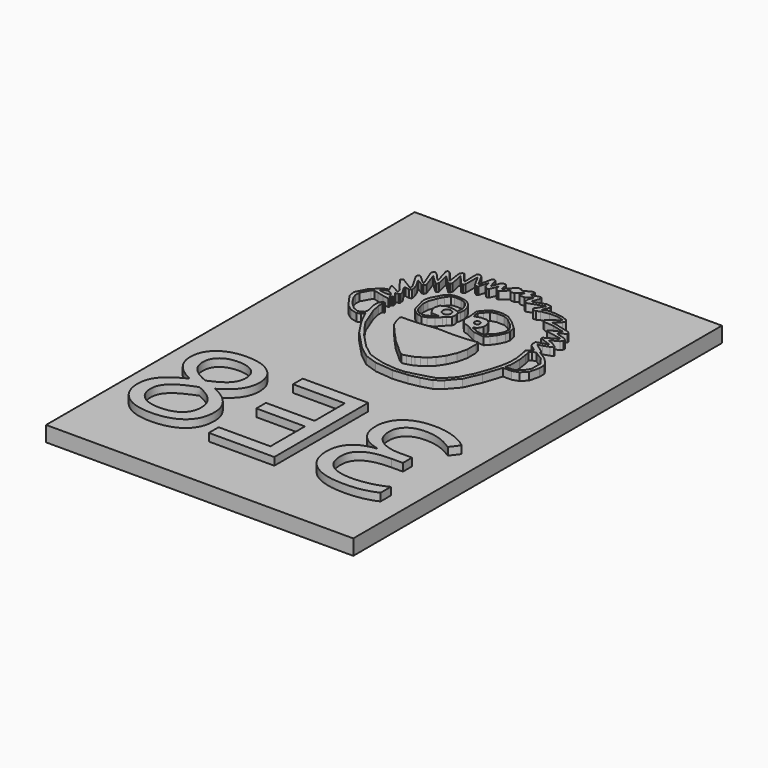
from build123d import *

# Parameters (mm, degrees)
F0_W         = 40
F0_H         = 60
F1_DEPTH     = 2
F2_TEXT_SIZE = 21.4073638846
F2_R         = 0.357844293
F2_R_2       = 0.5523242162
F3_DEPTH     = 3
F5_ANGLE     = 180


# Not quite as in the source:
# - Text() gives the source's letters only with a copy of the font that has no kerning and outlines rounded to 1/6400 em; it was checked with that copy


with BuildPart() as f1:
    # F0 (on Top) → F1 (new body)
    with BuildSketch(Plane.XY):
        Rectangle(F0_W, F0_H)
    extrude(amount=-F1_DEPTH)

    # F2 (on face) → F3 (join)
    with BuildSketch(Plane(origin=(0, 0, -2), x_dir=(1, 0, 0), z_dir=(0, 0, -1))):
        Polygon((-9.189459689, 13.5348810488), (-9.2555044294, 13.4181681694), (-10.3975787834, 12.584762522), (-10.4901792556, 12.3069606395), (-11.5087863133, 11.6587564023), (-12.1261237264, 11.0722858132), (-12.558260195, 10.424081576), (-12.558260195, 9.5906761614), (-12.2495910228, 8.3251342782), (-11.5705199614, 7.6151965092), (-10.7371147797, 7.3373945103), (-9.6259072498, 7.3373945103), (-8.8542347849, 4.9915125034), (-7.9282291308, 2.892565322), (-6.6935543046, 1.4726890856), (-5.7675486505, 0.7627512002), (-4.3785387725, 0.3614815557), (-3.0540523194, 0.0964602129), (-1.1776926304, -0.0722013741), (1.2046519941, 0.1597081916), (2.8912674561, 0.7289409311), (4.4724697172, 1.9728200184), (6.6861522309, 4.3129990715), (7.9932792969, 6.3158551108), (8.6257604807, 7.6018992019), (8.8155044168, 8.0235530529), (9.1317452416, 7.6440645987), (9.5744810924, 7.4543205462), (10.4388723075, 7.6862299954), (11.2610969618, 8.2765453168), (12.504976049, 10.0264091649), (12.6525543555, 10.8907999144), (11.8935786113, 12.3665881017), (11.2610969618, 12.9498689109), (10.7947986498, 13.3703084336), (10.322515659, 13.5592216299), (10.1808307618, 13.5592216299), (10.5303207338, 14.3337667593), (10.4219816507, 14.382651481), (9.6046447679, 13.9559403667), (9.3968396932, 13.7670267047), (9.1512517929, 13.7670267047), (9.302383095, 14.1920818621), (9.9541338086, 14.9855184042), (10.690847218, 15.9883339563), (10.3991904993, 16.2025981001), (8.8826266974, 15.2650455618), (8.7546797395, 15.3171446779), (8.8031513542, 15.6388244265), (9.8634593114, 17.4857479194), (9.8634593114, 17.788693183), (9.7230512574, 17.901346893), (9.4896217733, 17.8499919036), (8.4695348441, 16.8905964726), (8.369159691, 16.8905964726), (8.369159691, 17.0469944039), (9.1667303741, 19.0665655443), (9.1088505387, 19.4099162379), (8.9197883308, 19.5366152236), (8.4184741527, 19.1508362674), (7.6857789345, 18.2866071024), (7.5817767456, 18.2866071024), (8.1641504466, 20.2886032545), (8.0856618397, 20.4456875705), (7.8857758008, 20.4456875705), (7.6628642082, 20.2821175241), (6.6878812313, 19.0010591083), (6.5792927444, 19.0010591083), (6.8152903504, 20.7254605972), (6.6392480321, 21.0585369402), (6.3932228759, 21.0585369402), (5.3943090997, 19.7659152233), (5.2640845924, 19.7659152233), (5.313896846, 20.6956349918), (5.313896846, 21.6737444186), (5.1276095137, 21.8378741899), (4.8515007756, 21.8378741899), (4.6102980077, 21.5991920465), (3.8448546938, 20.1628588745), (3.7508065251, 20.2129785426), (3.4124271869, 21.8915016064), (3.1986572239, 21.9903782615), (2.9369632639, 21.7998669156), (2.6018317248, 20.5726175242), (2.1652462119, 21.6910027572), (1.9358477779, 21.8655924288), (1.7066724058, 21.8655924288), (1.5171964578, 21.7885960498), (1.3179039042, 20.8237523818), (0.2019009071, 22.0263794669), (-0.2691809978, 22.0263794669), (-0.4132577642, 21.83376892), (-0.4132577642, 21.7485696682), (-1.608875541, 22.3511316487), (-1.8950914573, 22.2474922099), (-1.8950914573, 22.0347762713), (-1.7497865092, 21.5740854525), (-2.8787629754, 21.9201136985), (-3.0722433776, 21.8083903798), (-3.0722433776, 21.4888442912), (-2.7170588337, 20.5106659466), (-3.5181820467, 20.785703198), (-4.3758560978, 21.0735172638), (-4.9409458488, 20.9864795813), (-5.1119194441, 20.6827808776), (-4.6780330204, 19.7794426837), (-5.303144183, 20.0162407615), (-6.4228956662, 20.0162407615), (-7.4601017013, 19.8396731773), (-8.0307817161, 19.5844498136), (-8.24605041, 19.3033533776), (-8.0752160475, 18.9340774575), (-7.4343785718, 18.3960458868), (-7.3064819053, 18.2485942402), (-7.8894097433, 18.1528887385), (-9.8450260312, 17.662368589), (-10.0632274598, 17.4525257805), (-10.0632274598, 17.2588265174), (-9.2694286332, 16.7433804506), (-9.2694286332, 16.6299444297), (-10.3714356274, 16.3117515528), (-10.7497630716, 16.0429821023), (-10.7497630716, 15.8157105231), (-10.5060694814, 15.5290242889), (-9.5397301093, 15.0264118471), (-9.5050336868, 14.9278080696), (-10.1310964236, 14.7075108581), (-10.7881587073, 14.2786650592), (-10.8735991717, 14.1022418299), (-10.4952348931, 13.9190028099), (-9.6939068362, 13.6496204556), (-9.3001715914, 13.5726396599), align=None)
        Polygon((-11.3430276588, 11.3477747561), (-10.1665381417, 12.0761071936), (-9.7184592933, 11.9456195877), (-9.4817701802, 11.6775998519), (-9.6478203386, 10.9875624673), (-9.8202779964, 9.7875330736), (-9.8202779964, 8.327060719), (-9.6632728428, 7.6724917068), (-10.7016285956, 7.6724917068), (-11.5608099923, 8.2125865062), (-12.0227627531, 8.9787616068), (-12.0227627531, 10.4255544626), align=None, mode=Mode.SUBTRACT)
        Polygon((-9.2021089122, 11.8955987179), (-9.6259845495, 12.3817160399), (-8.7710965499, 13.0297950142), (-8.6582891718, 13.3749520079), (-8.6582891718, 13.83907801), (-10.1395716965, 14.2732391739), (-8.597789526, 14.8448477173), (-8.6321562603, 15.0500525394), (-8.8547609821, 15.1859855884), (-10.0988355736, 15.8662788417), (-10.1283473969, 16.0429821023), (-8.1280890927, 16.3770521664), (-8.0309549421, 16.4534951234), (-8.0309549421, 16.6605234751), (-9.3255780712, 17.2988389292), (-9.3255780712, 17.4198456713), (-9.1570152045, 17.4198456713), (-7.8610751853, 17.7576577896), (-6.6900786087, 17.8401813516), (-6.3190494739, 18.0482565099), (-6.3680035137, 18.2607452059), (-7.6723454595, 19.1558197745), (-7.7717725262, 19.3576820799), (-6.9919994176, 19.5941383624), (-5.8549048454, 19.5941383624), (-4.8648479469, 19.4219628954), (-4.4465760775, 19.1960696736), (-4.0711632073, 19.1960696736), (-3.8452727795, 19.4726091483), (-4.5987849198, 20.6631215894), (-2.4533390142, 19.9265553289), (-2.2179344278, 20.1073296973), (-2.2179344278, 20.7775569194), (-2.4591403605, 21.2532266278), (-2.3988887742, 21.3428641343), (-1.6459601075, 20.8367685461), (-0.9518933557, 20.8367685461), (-0.805045439, 21.019308702), (-1.0992089397, 21.5109431249), (-1.0195223922, 21.5961252013), (-0.2568764803, 20.8826814554), (0.2120201406, 20.8826814554), (0.3918342218, 21.084864498), (1.3117186418, 20.2667534956), (1.5177458217, 20.2667534956), (1.7740993453, 20.4911687085), (1.8939064275, 21.0153785208), (2.3163190735, 20.022345581), (2.6061288472, 19.9079726496), (2.9661786202, 20.2604381972), (3.1901370194, 20.9794900053), (3.5305980518, 19.7691152477), (3.7267443649, 19.6868980908), (4.0454394575, 19.8750336328), (4.8510113656, 21.3132694968), (4.8510113656, 19.3455516034), (5.0149255357, 19.1363542014), (5.2653525881, 19.1363542014), (6.4009947628, 20.4648094856), (6.0275097303, 18.7064808467), (6.1335333548, 18.439371013), (6.3022564091, 18.3301762351), (7.5222377591, 19.5092194387), (7.1205476224, 17.8356234589), (7.2578334175, 17.6346850255), (7.4274286553, 17.6533626997), (8.5592081696, 18.700335049), (7.8939602636, 16.7839758703), (8.0356148928, 16.4933296525), (8.2925388515, 16.4933296525), (9.1843039208, 17.0311035363), (8.6411859765, 16.0850601875), (8.3799024969, 15.3487844997), (8.3799024969, 15.0033094594), (8.5981579423, 14.851562553), (9.1992679909, 14.9908660584), (9.275292784, 14.8559425631), (9.1386919766, 14.569966928), (8.7421050221, 13.9571603992), (8.6583698094, 13.5250080982), (8.8074074983, 13.3611097605), (9.3035807758, 13.3611097605), (9.0055147111, 13.0921600991), (8.8328046649, 12.7726279804), (8.8328046649, 12.5881325127), (9.010963068, 12.5194479616), (9.1582264676, 12.3547840537), (8.9850995676, 12.1999519706), (8.9941497817, 11.9886224763), (9.1404642835, 11.9948884146), (9.803073287, 12.1258817287), (10.623873949, 12.3241915041), (11.2366292551, 12.4787016445), (11.5004207864, 12.2345046745), (12.1156934574, 11.1478128144), (12.1156934574, 10.499742222), (11.9622180164, 9.9955123057), (11.2739799469, 8.9259134745), (10.4609073996, 8.1680297059), (9.7701705917, 7.8610534453), (9.4209367335, 7.9873521951), (9.1028444394, 8.1669735861), (8.9708127007, 8.5515753505), (9.0506223887, 8.9722721511), (9.204881072, 9.5914580067), (9.2938465923, 10.2266588853), (9.2200411409, 10.6872914964), (9.0513963178, 10.9562481427), (8.8901601657, 11.0822765761), (8.7422074675, 11.0587918804), (8.550712645, 10.8786210091), (8.5594270304, 10.7580808596), (8.6830591708, 10.740066287), (8.7972700521, 10.740066287), (8.7972700521, 10.0910024391), (8.5443880334, 8.9049179712), (8.1242027618, 7.8653744328), (7.5713287033, 6.4385982311), (6.6861522309, 5.1533160055), (5.8046395816, 4.0356008009), (4.1952138226, 2.3478454584), (2.7228207718, 1.228510742), (1.6501371674, 0.8664269605), (0.5779551238, 0.5780266271), (-0.5085729254, 0.456186817), (-1.3347239774, 0.3945332625), (-2.4423787445, 0.4550575883), (-3.9167545811, 0.8341207774), (-5.5857125744, 1.3082342827), (-6.3966686912, 1.8832468101), (-7.3317719698, 2.9245937382), (-8.1612218246, 4.5228650467), (-8.7279576883, 6.1055318126), (-9.1673780307, 7.5941767915), (-9.3645185307, 8.7970305373), (-9.3645185307, 9.8288155766), (-9.2588907182, 10.5280371988), (-9.1195667237, 11.3835189165), (-9.0252330601, 11.7312156269), align=None, mode=Mode.SUBTRACT)
        Polygon((9.5603252399, 13.0371160598), (9.8843954429, 13.2374589936), (10.1001633256, 13.2788474345), (10.5121981278, 13.1799288699), (10.7520677075, 13.0064216116), (10.8275951743, 12.8346410253), (10.531334944, 12.7722703525), (9.9573207944, 12.6837141485), (9.5230515972, 12.7355725178), (9.3631798327, 12.8573070885), align=None, mode=Mode.SUBTRACT)
        with Locations((-18.0694767914, -22.5213780068)):
            Text('3E8', F2_TEXT_SIZE, font='Open Sans', text_align=(TextAlign.LEFT, TextAlign.BOTTOM))
        Polygon((-2.5932078324, 9.9378599459), (-4.112102285, 10.137641211), (-4.2508884408, 9.6318180346), (-4.2508884408, 8.2489791), (-3.955797486, 6.9681084621), (-3.4152941853, 5.7855350512), (-2.8328874223, 4.9387547094), (-2.2081053278, 4.3190151991), (-1.5957122278, 3.9136625034), (-1.1420036128, 3.6378370204), (-0.7815588806, 3.4961389517), (-0.2557291111, 3.3374889826), (0.1739065001, 3.2302179513), (0.3918342218, 3.2689726119), (0.9345906246, 3.6690056929), (1.5618625721, 4.2602275404), (2.2558979297, 4.8684978464), (2.7284528667, 5.3091954978), (3.2852092217, 5.9283885109), (4.0007627494, 6.6972817201), (4.986223571, 7.8703290689), (5.3999910988, 8.9265593467), (5.4964109249, 9.4528837269), (5.4245561287, 9.5860982453), (3.4754090402, 9.6415715431), (0.915597232, 9.9233951093), (-1.0267217485, 9.8763281619), align=None)
        Polygon((-2.1723929867, 16.6633695969), (-2.9941883013, 16.4811814809), (-3.9514216669, 15.8269059518), (-5.0155857653, 14.860567511), (-5.231388107, 13.9517475524), (-5.1017587148, 13.399936133), (-4.6788586378, 12.5413465918), (-4.2540195473, 11.9674516515), (-3.7715008557, 11.4688746305), (-2.396504434, 11.6344543712), (-1.0310241096, 12.3511621402), (-0.3819549065, 12.5246605509), (0.0503193105, 13.0420954571), (0.1300272515, 13.5537449875), (0.0762266672, 14.04781627), (0.2374199203, 15.27546613), (0.0723192743, 15.584278726), (-0.5345819709, 16.2360415467), (-1.0026836144, 16.5532434964), (-1.5766988117, 16.6633695969), align=None)
        Polygon((-0.1165750628, 14.7014631563), (-0.2550073159, 14.3229745933), (-0.8960224996, 14.5691278064), (-1.7319852095, 14.5779129722), (-2.2096724324, 14.2550364741), (-2.4325162713, 13.7577265174), (-2.4314398952, 13.1487640226), (-2.2201318834, 12.7197567978), (-1.9343653303, 12.4825419531), (-1.7724684049, 12.4704310344), (-1.7102676984, 12.396911499), (-1.7475855611, 12.2880044998), (-1.9782550708, 12.1759254159), (-2.3868969104, 11.9888812841), (-2.8266529162, 11.8933775136), (-3.1929185689, 11.8191562266), (-3.5008960013, 11.8640306079), (-4.4143565074, 12.7688402915), (-4.7701496706, 13.4648060099), (-4.9055812024, 14.2937785619), (-4.2933744453, 15.1877588266), (-3.2846883014, 15.9890929842), (-2.6140033342, 16.2630992615), (-1.6628834028, 16.2843315535), (-0.948295773, 16.0998616972), (-0.5027595516, 15.5382760474), (-0.1036080839, 15.070862011), align=None, mode=Mode.SUBTRACT)
        with Locations((-1.3843593961, 13.4500422188)):
            Circle(F2_R, mode=Mode.SUBTRACT)
        Polygon((1.3897048002, 14.2145490879), (1.4955032775, 13.7759790429), (1.3754680212, 13.3076755935), (1.44481593, 12.8413940453), (1.8575723907, 12.5119726778), (2.1335671581, 12.2160956868), (2.6614377666, 11.6326211625), (3.3475812915, 11.2160452315), (3.8980571944, 10.9935378329), (4.4548309333, 11.1040746467), (4.8146828003, 11.2889216886), (5.377754841, 11.7325027147), (5.6196123287, 12.3399951169), (5.7611589245, 13.0087415361), (5.9384720325, 13.6048718029), (5.9984850622, 14.1340073803), (5.7975801565, 14.8063533613), (5.3796086386, 15.5532209807), (5.1052549779, 16.0898835072), (4.737034712, 16.4509442308), (4.2349321693, 16.6769566619), (3.7436595112, 16.718240329), (3.1430330518, 16.6763922804), (2.4245591294, 16.4872872317), (1.8735466683, 16.0395660111), (1.5190454824, 15.4573375964), (1.3410480269, 14.7608806053), align=None)
        with Locations((2.4974290672, 13.3780193188)):
            Circle(F2_R_2, mode=Mode.SUBTRACT)
        Polygon((2.1974599613, 14.2699516052), (1.76839092, 14.1540587553), (1.6981912004, 14.913517856), (1.9746389398, 15.6931689614), (2.4569535553, 16.1895108083), (3.1037636027, 16.3751513371), (3.9679916035, 16.3960939878), (4.3323885575, 16.2988536665), (4.7341545969, 15.7875491911), (5.1109779551, 15.0563249969), (5.4991979077, 14.0314063662), (5.5442338735, 13.3672495046), (5.4463374354, 12.8113444568), (5.2143882885, 12.0803936058), (5.0212180167, 11.7598435515), (4.5457210317, 11.4395030448), (3.9612055216, 11.3684468576), (3.3014659229, 11.6317904228), (2.8467637412, 11.9260646076), (2.5995469577, 12.2043726639), (3.2416775748, 12.200381481), (3.6520332023, 12.303595771), (3.9483793471, 12.736102906), (4.146346163, 13.3543697791), (3.962479338, 13.9931923383), (3.4327460844, 14.3504718923), (2.7684416082, 14.3502604821), align=None, mode=Mode.SUBTRACT)
    extrude(amount=-F3_DEPTH)


with BuildPart() as f1_1:
    # F4: moved
    add(f1.part.moved(Location((0, 0, 2))))


with BuildPart() as f1_2:
    # F5: moved
    add(f1_1.part.rotate(Axis((-1.1776926304, 0.0722013741, 1.5), (0, 0, -1)), F5_ANGLE))


solid = f1_2.part
